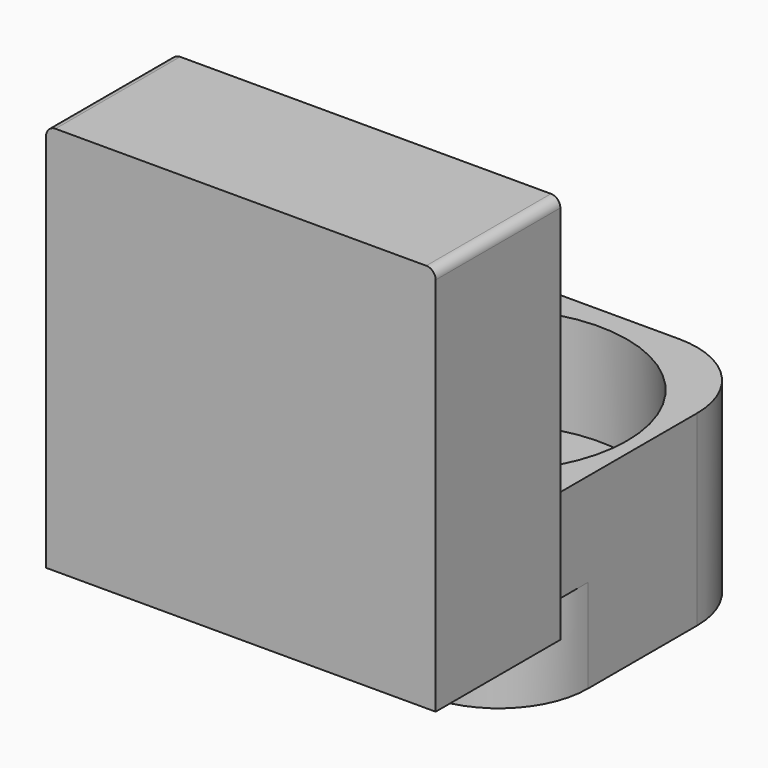
from build123d import *

# Parameters (mm, degrees)
F0_W     = 304.8
F0_H     = 121.92
F1_DEPTH = 304.8
F2_W     = 236.021310091
F2_H     = 246.3743686676
F3_DEPTH = 73.152
F4_R     = 69.9059679121
F5_R     = 107.4455989459
F6_DEPTH = 79.248
F7_R     = 7.3585229381
F8_W     = 48.9512532949
F8_H     = 10.1278424263
F9_DEPTH = 10.668


with BuildPart() as f1:
    # F0 (on Top) → F1 (new body)
    with BuildSketch(Plane.XY):
        with Locations((152.4, -60.96)):
            Rectangle(F0_W, F0_H)
    extrude(amount=F1_DEPTH)

    # F2 (on Top) → F3 (join, symmetric)
    with BuildSketch(Plane.XY):
        with Locations((152.538523078, 123.1871843338)):
            Rectangle(F2_W, F2_H)
    extrude(amount=F3_DEPTH, both=True)

    # F4
    f4_edges = [f1.edges().sort_by_distance(p)[0] for p in [
        (34.527868, 246.374369, 0),
        (270.549178, 246.374369, 0),
        (34.527868, 0, -36.576),
        (270.549178, 0, -36.576),
    ]]
    fillet(f4_edges, radius=F4_R)

    # F5 (on face) → F6 (cut)
    with BuildSketch(Plane.XY.offset(73.152)):
        with Locations((152.538523078, 121.3710904121)):
            Circle(F5_R)
    extrude(amount=-F6_DEPTH, mode=Mode.SUBTRACT)

    # F7
    f7_edges = [f1.edges().sort_by_distance(p)[0] for p in [
        (304.8, -60.96, 304.8),
        (0, -60.96, 304.8),
    ]]
    fillet(f7_edges, radius=F7_R)

    # F8 (on face) → F9 (join)
    with BuildSketch(Plane(origin=(0, 0, 0), x_dir=(-1, 0, 0), z_dir=(0, 1, 0))):
        with Locations((-264.9517431855, 283.5146784782)):
            Rectangle(F8_W, F8_H)
    extrude(amount=F9_DEPTH)


solid = f1.part
